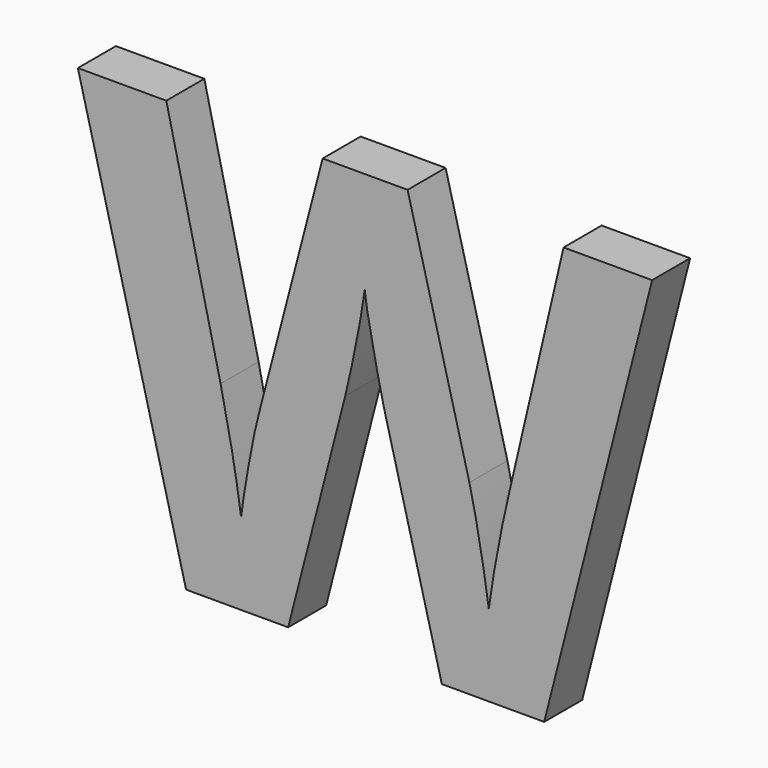
from build123d import *

# Parameters (mm, degrees)
F0_TEXT_SIZE = 62.5
F1_DEPTH     = 5


# Not quite as in the source:
# - Text() gives the source's letters only with a copy of the font that has no kerning and outlines rounded to 1/6400 em; it was checked with that copy


with BuildPart() as f1:
    # F0 (on Front) → F1 (new body)
    with BuildSketch(Plane.XZ):
        with Locations((-53.8902429503, 11.1951222276)):
            Text('W', F0_TEXT_SIZE, font='Open Sans', font_style=FontStyle.BOLD, text_align=(TextAlign.LEFT, TextAlign.BOTTOM))
    extrude(amount=F1_DEPTH)


solid = f1.part
